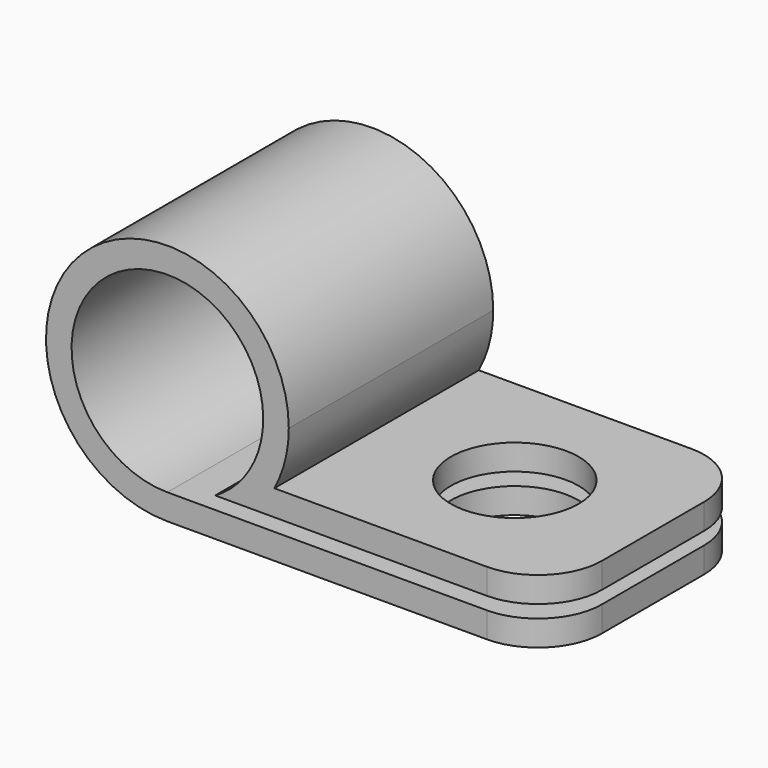
from build123d import *

# Parameters (mm, degrees)
F1_DEPTH = 8
F2_R     = 2
F3_DEPTH = 25
F4_R     = 2


# Not quite as in the source:
# - a feature names something its author has since deleted; it is built from what else it names


with BuildPart() as f1:
    # F0 (on Front) → F1 (new body)
    with BuildSketch(Plane.XZ):
        with BuildLine():
            ThreePointArc((0, -3), (-2.1213203436, 2.1213203436), (3, 0))
            ThreePointArc((3, 0), (2.8460498942, -0.9486832981), (2.4, -1.8))
            Line((2.4, -1.8), (3.3466401061, -1.8))
            ThreePointArc((3.3466401061, -1.8), (3.6849173941, -0.9281076437), (3.8, 0))
            ThreePointArc((3.8, 0), (-2.6870057685, 2.6870057685), (0, -3.8))
            Line((0, -3.8), (0, -3))
        make_face()
        with BuildLine():
            Line((2.3323807579, -3), (0, -3))
            Line((0, -3), (0, -3.8))
            ThreePointArc((0, -3.8), (1.2328828006, -3.5944401511), (2.3323807579, -3))
        make_face()
        with BuildLine():
            Line((3.3466401061, -1.8), (2.4, -1.8))
            ThreePointArc((2.4, -1.8), (1.9889684627, -2.2458861178), (1.4966629547, -2.6))
            Line((1.4966629547, -2.6), (2.7712812921, -2.6))
            ThreePointArc((2.7712812921, -2.6), (3.0850025217, -2.2187292402), (3.3466401061, -1.8))
        make_face()
        with BuildLine():
            Line((12, -3), (2.3323807579, -3))
            ThreePointArc((2.3323807579, -3), (1.2328828006, -3.5944401511), (0, -3.8))
            Line((0, -3.8), (12, -3.8))
            Line((12, -3.8), (12, -3))
        make_face()
        with BuildLine():
            Line((12, -1.8), (3.3466401061, -1.8))
            ThreePointArc((3.3466401061, -1.8), (3.0850025217, -2.2187292402), (2.7712812921, -2.6))
            Line((2.7712812921, -2.6), (12, -2.6))
            Line((12, -2.6), (12, -1.8))
        make_face()
    extrude(amount=F1_DEPTH)

    # F2 (on face) → F3 (cut)
    with BuildSketch(Plane.XY.offset(-1.8)):
        with Locations((7.6733200531, -4)):
            Circle(F2_R)
    extrude(amount=-F3_DEPTH, mode=Mode.SUBTRACT)

    # F4
    f4_edges = [f1.edges().sort_by_distance(p)[0] for p in [
        (12, -8, -2.2),
        (12, -8, -3.4),
        (12, 0, -3.4),
        (12, 0, -2.2),
    ]]
    fillet(f4_edges, radius=F4_R)


solid = f1.part
